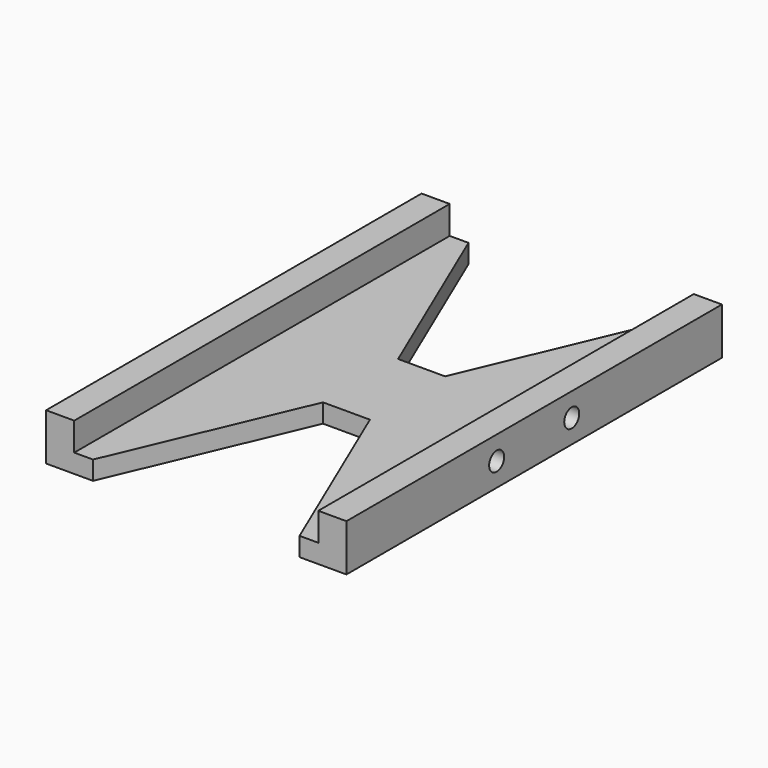
from build123d import *

# Parameters (mm, degrees)
F0_W     = 32
F0_H     = 50
F1_DEPTH = 5
F3_DEPTH = 5
F4_R     = 1
F5_DEPTH = 2.9
F7_DEPTH = 3


# Not quite as in the source:
# - a pattern or mirror of a feature is missing from the dataset's text; its kind, count and spacing are read off the source's solid


with BuildPart() as f1:
    # F0 (on Top) → F1 (new body)
    with BuildSketch(Plane.XY):
        Rectangle(F0_W, F0_H)
    extrude(amount=F1_DEPTH)

    # F2 (on face) → F3 (cut, through all)
    with BuildSketch(Plane.XY.offset(5)):
        Polygon((11, 25), (-11, 25), (-2.5, 5), (0, 5), (2.5, 5), align=None)
        Polygon((0, -5), (-2.5, -5), (-11, -25), (11, -25), (2.5, -5), align=None)
    extrude(amount=-F3_DEPTH, mode=Mode.SUBTRACT)

    # F4 (on face) → F5 (cut)
    with BuildSketch(Plane(origin=(-16, 0, 0), x_dir=(0, -1, 0), z_dir=(-1, 0, 0))):
        with Locations((-5, 2.5)):
            Circle(F4_R)
        with Locations((5, 2.5)):
            Circle(F4_R)
    f5 = extrude(amount=-F5_DEPTH, mode=Mode.SUBTRACT)

    # F5_copies: F5 across plane
    add(f5.mirror(Plane(origin=(0, 0, 0), x_dir=(0, 0, 1), z_dir=(1, 0, 0))), mode=Mode.SUBTRACT)

    # F6 (on face) → F7 (cut)
    with BuildSketch(Plane.XY.offset(5)):
        Polygon((-11, 25), (-13, 25), (-13, -25), (-11, -25), (-2.5, -5), (2.5, -5), (11, -25), (13, -25), (13, 25), (11, 25), (2.5, 5), (-2.5, 5), align=None)
    extrude(amount=-F7_DEPTH, mode=Mode.SUBTRACT)


solid = f1.part
